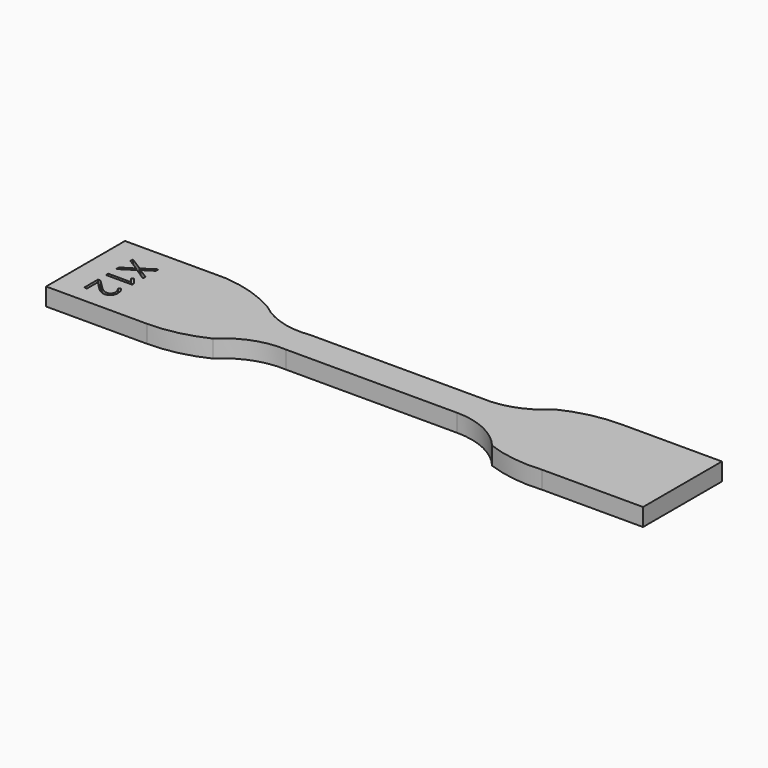
from build123d import *

# Parameters (mm, degrees)
F1_DEPTH     = 3.4
F2_TEXT_SIZE = 7.0564552314
F3_DEPTH     = 1


# Not quite as in the source:
# - Text() gives the source's letters only with a copy of the font that has no kerning and outlines rounded to 1/6400 em; it was checked with that copy


with BuildPart() as f1:
    # F0 (on Top) → F1 (new body)
    with BuildSketch(Plane.XY):
        with BuildLine():
            Line((-14.4320548165, 19.7811394548), (-33.8720548165, 19.7811394548))
            Line((-33.8720548165, 19.7811394548), (-33.8720548165, 0.7811394548))
            Line((-33.8720548165, 0.7811394548), (-14.4320548165, 0.7811394548))
            ThreePointArc((-14.4320548165, 0.7811394548), (-8.9053122052, 1.3996892086), (-3.6520548165, 3.2247301661))
            ThreePointArc((-3.6520548165, 3.2247301661), (1.3014698263, 6.4128780055), (7.1279451835, 7.2811394548))
            Line((7.1279451835, 7.2811394548), (40.1279451835, 7.2811394548))
            ThreePointArc((40.1279451835, 7.2811394548), (46.0837574042, 5.9511158081), (50.9079451835, 2.2137538538))
            ThreePointArc((50.9079451835, 2.2137538538), (56.2191047011, 0.9041953221), (61.6879451835, 0.7811394548))
            Line((61.6879451835, 0.7811394548), (81.1279451835, 0.7811394548))
            Line((81.1279451835, 0.7811394548), (81.1279451835, 19.7811394548))
            Line((81.1279451835, 19.7811394548), (61.6879451835, 19.7811394548))
            ThreePointArc((61.6879451835, 19.7811394548), (56.1612025723, 19.162589701), (50.9079451835, 17.3375487435))
            ThreePointArc((50.9079451835, 17.3375487435), (45.9544205407, 14.1494009041), (40.1279451835, 13.2811394548))
            Line((40.1279451835, 13.2811394548), (7.1279451835, 13.2811394548))
            ThreePointArc((7.1279451835, 13.2811394548), (1.4167452884, 13.6925537245), (-3.6520548165, 16.3560723447))
            ThreePointArc((-3.6520548165, 16.3560723447), (-8.8458057958, 18.686276846), (-14.4320548165, 19.7811394548))
        make_face()
    extrude(amount=F1_DEPTH)

    # F2 (on face) → F3 (cut)
    with BuildSketch(Plane.XY.offset(3.4)):
        with Locations(Location((-29.1824135929, 15.8650862949), (0, 0, -90))):
            Text('X12', F2_TEXT_SIZE, font='Open Sans', text_align=(TextAlign.LEFT, TextAlign.BOTTOM))
    extrude(amount=-F3_DEPTH, mode=Mode.SUBTRACT)


solid = f1.part
